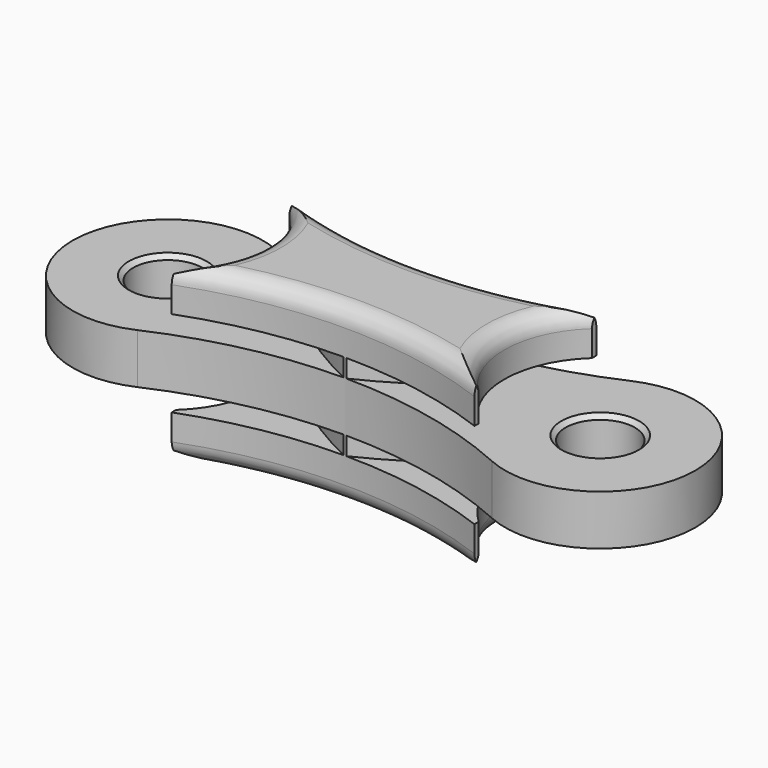
from build123d import *

# Parameters (mm, degrees)
F1_DEPTH      = 10
F2_W          = 35
F2_H          = 12.1
F3_DEPTH      = 12.5
F4_R          = 11.1
F5_DEPTH      = 10
F6_R          = 11.1
F7_DEPTH      = 10
F9_T2_ANGLE   = 146.6276322734
F9_T4_ANGLE   = 146.6276322734
F9_T6_ANGLE   = 52.4347400512
F9_T8_ANGLE   = 52.4347400512
F9_T10_ANGLE  = 146.6276322734
F9_T12_ANGLE  = 146.6276322734
F9_T14_ANGLE  = 52.4347400512
F9_T16_ANGLE  = 52.4347400512
F10_R         = 4
F11_DEPTH     = 12.9010001
F13_R         = 11
F14_DEPTH     = 2.1
F12_R         = 11
F15_DEPTH     = 2.1
F16_SIZE      = 0.5
F17_TEXT_SIZE = 2.8660994178
F18_DEPTH     = 0.2


# Not quite as in the source:
# - a fillet or chamfer that OpenCascade refuses, or shapes differently, is made with other operations: its cross-section is extruded or revolved along the edge and cut away or added
# - Text() gives the source's letters only with a copy of the font that has no kerning and outlines rounded to 1/6400 em; it was checked with that copy


with BuildPart() as f1:
    # F0 (on Top) → F1 (new body, symmetric)
    with BuildSketch(Plane.XY):
        with BuildLine():
            ThreePointArc((20.4918032787, 10.0337511591), (0, 5.641710973), (-20.4918032787, 10.0337511591))
            ThreePointArc((-20.4918032787, 10.0337511591), (-36, 0), (-20.4918032787, -10.0337511591))
            ThreePointArc((-20.4918032787, -10.0337511591), (0, -5.641710973), (20.4918032787, -10.0337511591))
            ThreePointArc((20.4918032787, -10.0337511591), (36, 0), (20.4918032787, 10.0337511591))
        make_face()
    extrude(amount=F1_DEPTH, both=True)

    # F2 (on Front) → F3 (cut, symmetric)
    with BuildSketch(Plane.XZ):
        with Locations((-35, 8.95)):
            Rectangle(F2_W, F2_H)
        with Locations((-35, -8.95)):
            Rectangle(F2_W, F2_H)
        with Locations((35, 8.95)):
            Rectangle(F2_W, F2_H)
        with Locations((35, -8.95)):
            Rectangle(F2_W, F2_H)
    extrude(amount=F3_DEPTH, both=True, mode=Mode.SUBTRACT)

    # F4 (on face) → F5 (cut)
    with BuildSketch(Plane.XY.offset(2.9)):
        with BuildLine():
            ThreePointArc((-17.5, -8.1829090182), (-14.8397834669, -4.4698993277), (-13.9, 0))
            ThreePointArc((-13.9, 0), (-14.8397834669, 4.4698993277), (-17.5, 8.1829090182))
            Line((-17.5, 8.1829090182), (-17.5, -8.1829090182))
        make_face()
        with BuildLine():
            Line((-17.5, -8.1829090182), (-17.5, 8.1829090182))
            ThreePointArc((-17.5, 8.1829090182), (-18.3457990647, 8.8843463414), (-19.2568056465, 9.4987219465))
            ThreePointArc((-19.2568056465, 9.4987219465), (-19.8761047979, 9.7620808735), (-20.4918032787, 10.0337511591))
            ThreePointArc((-20.4918032787, 10.0337511591), (-36, 0), (-20.4918032787, -10.0337511591))
            ThreePointArc((-20.4918032787, -10.0337511591), (-19.8761047979, -9.7620808735), (-19.2568056465, -9.4987219465))
            ThreePointArc((-19.2568056465, -9.4987219465), (-18.3457990647, -8.8843463414), (-17.5, -8.1829090182))
        make_face()
        with Locations((25, 0)):
            Circle(F4_R)
    extrude(amount=F5_DEPTH, mode=Mode.SUBTRACT)

    # F6 (on face) → F7 (cut)
    with BuildSketch(Plane(origin=(0, 0, -2.9), x_dir=(1, 0, 0), z_dir=(0, 0, -1))):
        with BuildLine():
            ThreePointArc((-17.5, -8.1829090182), (-14.8397834669, -4.4698993277), (-13.9, 0))
            ThreePointArc((-13.9, 0), (-14.8397834669, 4.4698993277), (-17.5, 8.1829090182))
            Line((-17.5, 8.1829090182), (-17.5, -8.1829090182))
        make_face()
        with BuildLine():
            Line((-17.5, -8.1829090182), (-17.5, 8.1829090182))
            ThreePointArc((-17.5, 8.1829090182), (-18.3457990647, 8.8843463414), (-19.2568056465, 9.4987219465))
            ThreePointArc((-19.2568056465, 9.4987219465), (-19.8761047979, 9.7620808735), (-20.4918032787, 10.0337511591))
            ThreePointArc((-20.4918032787, 10.0337511591), (-36, 0), (-20.4918032787, -10.0337511591))
            ThreePointArc((-20.4918032787, -10.0337511591), (-19.8761047979, -9.7620808735), (-19.2568056465, -9.4987219465))
            ThreePointArc((-19.2568056465, -9.4987219465), (-18.3457990647, -8.8843463414), (-17.5, -8.1829090182))
        make_face()
        with Locations((25, 0)):
            Circle(F6_R)
    extrude(amount=F7_DEPTH, mode=Mode.SUBTRACT)

    # F9: fillet of radius 2 on 8 edges, made by hand

    # F9_s1 → F9_t2 (revolve, cut)
    with BuildSketch(Plane(origin=(-22.93891561, -6.8759756317, 0), x_dir=(0, 0, 1), z_dir=(-0.9578917603, -0.287129545, 0))):
        with BuildLine():
            ThreePointArc((-10, -5.9217613754), (-9.4142135624, -4.5075478131), (-8, -3.9217613754))
            Line((-8, -3.9217613754), (-10, -3.9217613754))
            Line((-10, -3.9217613754), (-10, -5.9217613754))
        make_face()
    revolve(axis=Axis((-25, 0, -10), (0, 0, 1)), revolution_arc=F9_T2_ANGLE, mode=Mode.SUBTRACT)

    # F9_s3 → F9_t4 (revolve, cut)
    with BuildSketch(Plane(origin=(22.93891561, 6.8759756317, 0), x_dir=(0, 0, 1), z_dir=(0.9578917603, 0.287129545, 0))):
        with BuildLine():
            ThreePointArc((-10, -5.9217613754), (-9.4142135624, -4.5075478131), (-8, -3.9217613754))
            Line((-8, -3.9217613754), (-10, -3.9217613754))
            Line((-10, -3.9217613754), (-10, -5.9217613754))
        make_face()
    revolve(axis=Axis((25, 0, -10), (0, 0, 1)), revolution_arc=F9_T4_ANGLE, mode=Mode.SUBTRACT)

    # F9_s5 → F9_t6 (revolve, cut)
    with BuildSketch(Plane(origin=(22.0524638961, 10.8594629696, 0), x_dir=(0, 0, 1), z_dir=(0.8971244797, 0.4417778491, 0))):
        with BuildLine():
            ThreePointArc((-10, 2.0824589936), (-9.4142135624, 0.6682454312), (-8, 0.0824589936))
            Line((-8, 0.0824589936), (-10, 0.0824589936))
            Line((-10, 0.0824589936), (-10, 2.0824589936))
        make_face()
    revolve(axis=Axis((0, 55.641710973, -10), (0, 0, -1)), revolution_arc=F9_T6_ANGLE, mode=Mode.SUBTRACT)

    # F9_s7 → F9_t8 (revolve, cut)
    with BuildSketch(Plane(origin=(-22.0524638961, -10.8594629696, 0), x_dir=(0, 0, 1), z_dir=(-0.8971244797, -0.4417778491, 0))):
        with BuildLine():
            ThreePointArc((-10, 2.0824589936), (-9.4142135624, 0.6682454312), (-8, 0.0824589936))
            Line((-8, 0.0824589936), (-10, 0.0824589936))
            Line((-10, 0.0824589936), (-10, 2.0824589936))
        make_face()
    revolve(axis=Axis((0, -55.641710973, -10), (0, 0, -1)), revolution_arc=F9_T8_ANGLE, mode=Mode.SUBTRACT)

    # F9_s9 → F9_t10 (revolve, cut)
    with BuildSketch(Plane(origin=(-22.93891561, 6.8759756317, 0), x_dir=(0, 0, 1), z_dir=(-0.9578917603, 0.287129545, 0))):
        with BuildLine():
            ThreePointArc((10, 5.9217613754), (9.4142135624, 4.5075478131), (8, 3.9217613754))
            Line((8, 3.9217613754), (10, 3.9217613754))
            Line((10, 3.9217613754), (10, 5.9217613754))
        make_face()
    revolve(axis=Axis((-25, 0, 10), (0, 0, -1)), revolution_arc=F9_T10_ANGLE, mode=Mode.SUBTRACT)

    # F9_s11 → F9_t12 (revolve, cut)
    with BuildSketch(Plane(origin=(22.93891561, -6.8759756317, 0), x_dir=(0, 0, 1), z_dir=(0.9578917603, -0.287129545, 0))):
        with BuildLine():
            ThreePointArc((10, 5.9217613754), (9.4142135624, 4.5075478131), (8, 3.9217613754))
            Line((8, 3.9217613754), (10, 3.9217613754))
            Line((10, 3.9217613754), (10, 5.9217613754))
        make_face()
    revolve(axis=Axis((25, 0, 10), (0, 0, -1)), revolution_arc=F9_T12_ANGLE, mode=Mode.SUBTRACT)

    # F9_s13 → F9_t14 (revolve, cut)
    with BuildSketch(Plane(origin=(22.0524638961, 10.8594629696, 0), x_dir=(0, 0, 1), z_dir=(0.8971244797, 0.4417778491, 0))):
        with BuildLine():
            ThreePointArc((10, 2.0824589936), (9.4142135624, 0.6682454312), (8, 0.0824589936))
            Line((8, 0.0824589936), (10, 0.0824589936))
            Line((10, 0.0824589936), (10, 2.0824589936))
        make_face()
    revolve(axis=Axis((0, 55.641710973, 10), (0, 0, -1)), revolution_arc=F9_T14_ANGLE, mode=Mode.SUBTRACT)

    # F9_s15 → F9_t16 (revolve, cut)
    with BuildSketch(Plane(origin=(-22.0524638961, -10.8594629696, 0), x_dir=(0, 0, 1), z_dir=(-0.8971244797, -0.4417778491, 0))):
        with BuildLine():
            ThreePointArc((10, 2.0824589936), (9.4142135624, 0.6682454312), (8, 0.0824589936))
            Line((8, 0.0824589936), (10, 0.0824589936))
            Line((10, 0.0824589936), (10, 2.0824589936))
        make_face()
    revolve(axis=Axis((0, -55.641710973, 10), (0, 0, -1)), revolution_arc=F9_T16_ANGLE, mode=Mode.SUBTRACT)

    # F10 (on face) → F11 (cut, through all)
    with BuildSketch(Plane(origin=(0, 0, -2.9), x_dir=(1, 0, 0), z_dir=(0, 0, -1))):
        with Locations((-25, 0)):
            Circle(F10_R)
        with Locations((25, 0)):
            Circle(F10_R)
    extrude(amount=-F11_DEPTH, mode=Mode.SUBTRACT)

    # F13 (on face) → F14 (cut)
    with BuildSketch(Plane(origin=(0, 0, -2.9), x_dir=(1, 0, 0), z_dir=(0, 0, -1))):
        with BuildLine():
            Line((0, 6.4569755857), (-13.1638717585, 16.1216025336))
            ThreePointArc((-13.1638717585, 16.1216025336), (-44.9999999952, 0.0004403993), (-13.1645817642, -16.1221237802))
            Line((-13.1645817642, -16.1221237802), (0, -6.4578678047))
            Line((0, -6.4578678047), (13.1645817642, -16.1221237802))
            ThreePointArc((13.1645817642, -16.1221237802), (44.9999999952, 0.0004403993), (13.1638717585, 16.1216025336))
            Line((13.1638717585, 16.1216025336), (0, 6.4569755857))
        make_face()
        with Locations((-25, 0)):
            Circle(F13_R, mode=Mode.SUBTRACT)
        with BuildLine():
            ThreePointArc((9.2058284956, 0.0126422507), (4.7571914607, -3.0803281815), (0, -5.6737751098))
            ThreePointArc((0, -5.6737751098), (-4.7571914607, -3.0803281815), (-9.2058284956, 0.0126422507))
            ThreePointArc((-9.2058284956, 0.0126422507), (-4.7578540322, 3.1153923915), (0, 5.7181525169))
            ThreePointArc((0, 5.7181525169), (4.7578540322, 3.1153923915), (9.2058284956, 0.0126422507))
        make_face(mode=Mode.SUBTRACT)
        with BuildLine():
            ThreePointArc((20.4918032787, 10.0337511591), (30.9753592388, 9.235533659), (36, 0))
            ThreePointArc((36, 0), (30.9753592388, -9.235533659), (20.4918032787, -10.0337511591))
            ThreePointArc((20.4918032787, -10.0337511591), (19.005846788, -9.3947890444), (17.5, -8.804225985))
            Line((17.5, -8.804225985), (17.5, -8.1829090182))
            ThreePointArc((17.5, -8.1829090182), (13.9, 0), (17.5, 8.1829090182))
            Line((17.5, 8.1829090182), (17.5, 8.804225985))
            ThreePointArc((17.5, 8.804225985), (19.005846788, 9.3947890444), (20.4918032787, 10.0337511591))
        make_face(mode=Mode.SUBTRACT)
    extrude(amount=F14_DEPTH, mode=Mode.SUBTRACT)

    # F12 (on face) → F15 (cut)
    with BuildSketch(Plane.XY.offset(2.9)):
        with BuildLine():
            Line((0, 6.4569755857), (-13.1638717585, 16.1216025336))
            ThreePointArc((-13.1638717585, 16.1216025336), (-44.9999999952, 0.0004403993), (-13.1645817642, -16.1221237802))
            Line((-13.1645817642, -16.1221237802), (0, -6.4578678047))
            Line((0, -6.4578678047), (13.1645817642, -16.1221237802))
            ThreePointArc((13.1645817642, -16.1221237802), (44.9999999952, 0.0004403993), (13.1638717585, 16.1216025336))
            Line((13.1638717585, 16.1216025336), (0, 6.4569755857))
        make_face()
        with BuildLine():
            ThreePointArc((0, -5.7181525169), (-4.7578540322, -3.1153923915), (-9.2058284956, -0.0126422507))
            ThreePointArc((-9.2058284956, -0.0126422507), (-4.7571914607, 3.0803281815), (0, 5.6737751098))
            ThreePointArc((0, 5.6737751098), (4.7571914607, 3.0803281815), (9.2058284956, -0.0126422507))
            ThreePointArc((9.2058284956, -0.0126422507), (4.7578540322, -3.1153923915), (0, -5.7181525169))
        make_face(mode=Mode.SUBTRACT)
        with BuildLine():
            ThreePointArc((-20.4918032787, -10.0337511591), (-36, 0), (-20.4918032787, 10.0337511591))
            ThreePointArc((-20.4918032787, 10.0337511591), (-19.005846788, 9.3947890444), (-17.5, 8.804225985))
            Line((-17.5, 8.804225985), (-17.5, 8.1829090182))
            ThreePointArc((-17.5, 8.1829090182), (-13.9, 0), (-17.5, -8.1829090182))
            Line((-17.5, -8.1829090182), (-17.5, -8.804225985))
            ThreePointArc((-17.5, -8.804225985), (-19.005846788, -9.3947890444), (-20.4918032787, -10.0337511591))
        make_face(mode=Mode.SUBTRACT)
        with Locations((25, 0)):
            Circle(F12_R, mode=Mode.SUBTRACT)
    extrude(amount=F15_DEPTH, mode=Mode.SUBTRACT)

    # F16
    f16_edges = [f1.edges().sort_by_distance(p)[0] for p in [
        (21, 0, -2.9),
        (-29, 0, -2.9),
        (21, 0, 2.9),
        (-29, 0, 2.9),
    ]]
    chamfer(f16_edges, length=F16_SIZE)

    # F17 (on face) → F18 (cut)
    with BuildSketch(Plane(origin=(0, 0, -10), x_dir=(1, 0, 0), z_dir=(0, 0, -1))):
        with Locations((-7.5, -1.0079881332)):
            Text('EMCEE.IND', F17_TEXT_SIZE, font='Open Sans', text_align=(TextAlign.LEFT, TextAlign.BOTTOM))
    extrude(amount=-F18_DEPTH, mode=Mode.SUBTRACT)


solid = f1.part
